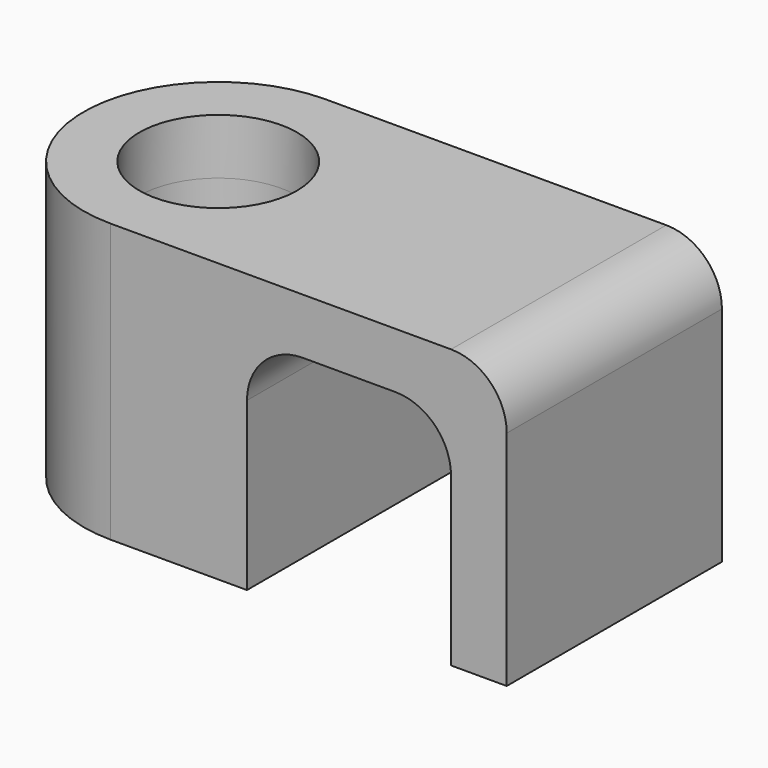
from build123d import *

# Parameters (mm, degrees)
F0_R        = 4.25
F0_W        = 11
F0_H        = 14.5
F0_W_2      = 3
F1_DEPTH    = 3
F2_DEPTH    = 12
F3_T1_DEPTH = 14.5
F3_T3_DEPTH = 29.5
F5_R        = 4.25
F6_DEPTH    = 22
F7_DEPTH    = 3
F8_T1_DEPTH = 28


# Not quite as in the source:
# - a fillet or chamfer that OpenCascade refuses, or shapes differently, is made with other operations: its cross-section is extruded or revolved along the edge and cut away or added


with BuildPart() as f1:
    # F0 (on Top) → F1 (new body)
    with BuildSketch(Plane.XY):
        with BuildLine():
            ThreePointArc((0, -7.25), (5.1265241636, -5.1265241636), (7.25, 0))
            ThreePointArc((7.25, 0), (5.1265241636, 5.1265241636), (0, 7.25))
            ThreePointArc((0, 7.25), (-7.25, 0), (0, -7.25))
        make_face()
        Circle(F0_R, mode=Mode.SUBTRACT)
        with BuildLine():
            Line((7.25, -7.25), (7.25, 0))
            ThreePointArc((7.25, 0), (5.1265241636, -5.1265241636), (0, -7.25))
            Line((0, -7.25), (7.25, -7.25))
        make_face()
        with BuildLine():
            ThreePointArc((0, 7.25), (5.1265241636, 5.1265241636), (7.25, 0))
            Line((7.25, 0), (7.25, 7.25))
            Line((7.25, 7.25), (0, 7.25))
        make_face()
        Polygon((7.25, 7.25), (7.25, 0), (7.25, -7.25), (7.35, -7.25), (7.35, 7.25), align=None)
        with Locations((12.85, 0)):
            Rectangle(F0_W, F0_H)
        with Locations((19.85, 0)):
            Rectangle(F0_W_2, F0_H)
    extrude(amount=F1_DEPTH)

    # F0 (on Top) → F2 (join)
    with BuildSketch(Plane.XY):
        with BuildLine():
            ThreePointArc((0, -7.25), (5.1265241636, -5.1265241636), (7.25, 0))
            ThreePointArc((7.25, 0), (5.1265241636, 5.1265241636), (0, 7.25))
            ThreePointArc((0, 7.25), (-7.25, 0), (0, -7.25))
        make_face()
        Circle(F0_R, mode=Mode.SUBTRACT)
        with BuildLine():
            ThreePointArc((0, 7.25), (5.1265241636, 5.1265241636), (7.25, 0))
            Line((7.25, 0), (7.25, 7.25))
            Line((7.25, 7.25), (0, 7.25))
        make_face()
        Polygon((7.25, 7.25), (7.25, 0), (7.25, -7.25), (7.35, -7.25), (7.35, 7.25), align=None)
        with Locations((19.85, 0)):
            Rectangle(F0_W_2, F0_H)
        with BuildLine():
            Line((7.25, -7.25), (7.25, 0))
            ThreePointArc((7.25, 0), (5.1265241636, -5.1265241636), (0, -7.25))
            Line((0, -7.25), (7.25, -7.25))
        make_face()
    extrude(amount=-F2_DEPTH)

    # F3: fillet of radius 3 on 3 edges, made by hand

    # F3_s2 → F3_t1 (join)
    with BuildSketch(Plane.XZ.offset(-7.25)):
        with BuildLine():
            ThreePointArc((7.35, -3), (8.2286796564, -0.8786796564), (10.35, 0))
            Line((10.35, 0), (7.35, 0))
            Line((7.35, 0), (7.35, -3))
        make_face()
        with BuildLine():
            ThreePointArc((15.35, 0), (17.4713203436, -0.8786796564), (18.35, -3))
            Line((18.35, -3), (18.35, 0))
            Line((18.35, 0), (15.35, 0))
        make_face()
    extrude(amount=F3_T1_DEPTH)

    # F3_s4 → F3_t3 (cut)
    with BuildSketch(Plane.XZ.offset(-14.75)):
        with BuildLine():
            ThreePointArc((18.35, 3), (20.4713203436, 2.1213203436), (21.35, 0))
            Line((21.35, 0), (21.35, 3))
            Line((21.35, 3), (18.35, 3))
        make_face()
    extrude(amount=F3_T3_DEPTH, mode=Mode.SUBTRACT)


with BuildPart() as f6:
    # F5 (on offset) → F6 (new body)
    with BuildSketch(Plane(origin=(0, 0, -37), x_dir=(1, 0, 0), z_dir=(0, 0, -1))):
        with BuildLine():
            Line((7.35, 7.25), (0, 7.25))
            ThreePointArc((0, 7.25), (-7.25, 0), (0, -7.25))
            Line((0, -7.25), (7.35, -7.25))
            Line((7.35, -7.25), (7.35, 7.25))
        make_face()
        Circle(F5_R, mode=Mode.SUBTRACT)
    extrude(amount=-F6_DEPTH)

    # F5 (on offset) → F7 (join)
    with BuildSketch(Plane(origin=(0, 0, -37), x_dir=(1, 0, 0), z_dir=(0, 0, -1))):
        with BuildLine():
            Line((7.35, 7.25), (0, 7.25))
            ThreePointArc((0, 7.25), (-7.25, 0), (0, -7.25))
            Line((0, -7.25), (7.35, -7.25))
            Line((7.35, -7.25), (7.35, 7.25))
        make_face()
        Circle(F5_R, mode=Mode.SUBTRACT)
        with BuildLine():
            ThreePointArc((0, -7.25), (-7.25, 0), (0, 7.25))
            Line((0, 7.25), (-37.25, 7.25))
            Line((-37.25, 7.25), (-37.25, 4))
            Line((-37.25, 4), (-22.25, 4))
            ThreePointArc((-22.25, 4), (-18.25, 0), (-22.25, -4))
            Line((-22.25, -4), (-37.25, -4))
            Line((-37.25, -4), (-37.25, -7.25))
            Line((-37.25, -7.25), (0, -7.25))
        make_face()
    extrude(amount=F7_DEPTH)

    # F8: fillet of radius 5 on 2 edges, made by hand

    # F8_s2 → F8_t1 (cut)
    with BuildSketch(Plane.XY.offset(-52.5)):
        with BuildLine():
            ThreePointArc((-32.25, -7.25), (-35.7855339059, -5.7855339059), (-37.25, -2.25))
            Line((-37.25, -2.25), (-37.25, -7.25))
            Line((-37.25, -7.25), (-32.25, -7.25))
        make_face()
        with BuildLine():
            ThreePointArc((-32.25, 7.25), (-35.7855339059, 5.7855339059), (-37.25, 2.25))
            Line((-37.25, 2.25), (-37.25, 7.25))
            Line((-37.25, 7.25), (-32.25, 7.25))
        make_face()
    extrude(amount=F8_T1_DEPTH, mode=Mode.SUBTRACT)


solid = f1.part
